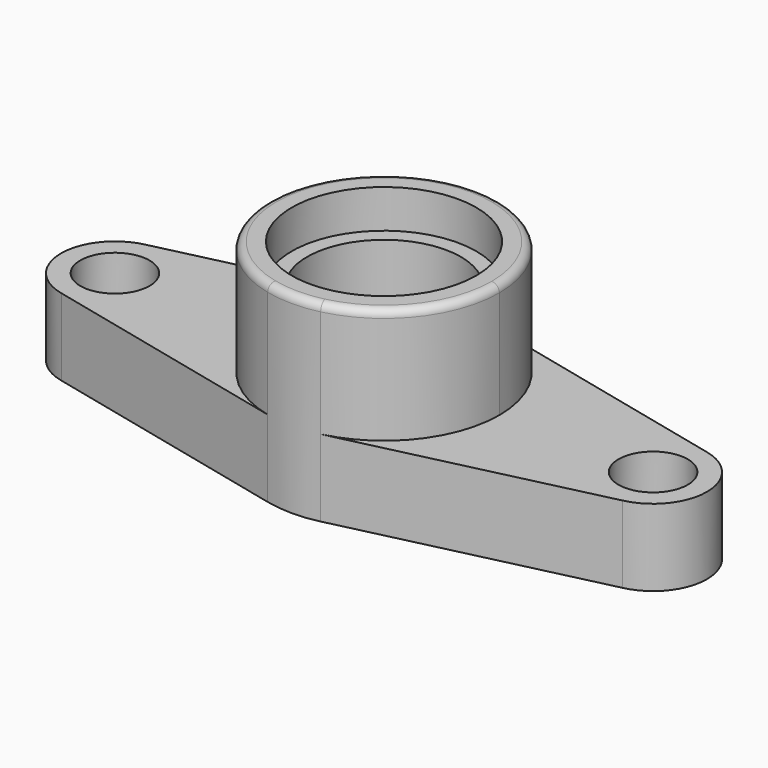
from build123d import *

# Parameters (mm, degrees)
F0_R     = 12
F0_R_2   = 4.5
F1_DEPTH = 10
F2_DEPTH = 25
F0_R_3   = 10
F3_DEPTH = 20
F0_R_4   = 3
F4_DEPTH = 5
F5_R     = 1


with BuildPart() as f1:
    # F0 (on Top) → F1 (new body)
    with BuildSketch(Plane.XY):
        with BuildLine():
            ThreePointArc((3.4443996306, -14.599181867), (11.761504888, -9.3095114142), (15, 0))
            ThreePointArc((15, 0), (11.761504888, 9.3095114142), (3.4443996306, 14.599181867))
            ThreePointArc((3.4443996306, 14.599181867), (0, 15), (-3.4443996306, 14.599181867))
            ThreePointArc((-3.4443996306, 14.599181867), (-15, 0), (-3.4443996306, -14.599181867))
            ThreePointArc((-3.4443996306, -14.599181867), (0, -15), (3.4443996306, -14.599181867))
        make_face()
        Circle(F0_R, mode=Mode.SUBTRACT)
        with BuildLine():
            ThreePointArc((3.4443996306, 14.599181867), (11.761504888, 9.3095114142), (15, 0))
            ThreePointArc((15, 0), (11.761504888, -9.3095114142), (3.4443996306, -14.599181867))
            Line((3.4443996306, -14.599181867), (36.4981958522, -6.8377927132))
            ThreePointArc((36.4981958522, -6.8377927132), (42, 0), (36.4981958522, 6.8377927132))
            Line((36.4981958522, 6.8377927132), (3.4443996306, 14.599181867))
        make_face()
        with Locations((35, 0)):
            Circle(F0_R_2, mode=Mode.SUBTRACT)
        with BuildLine():
            ThreePointArc((-3.4443996306, -14.599181867), (-15, 0), (-3.4443996306, 14.599181867))
            Line((-3.4443996306, 14.599181867), (-36.4981958522, 6.8377927132))
            ThreePointArc((-36.4981958522, 6.8377927132), (-42, 0), (-36.4981958522, -6.8377927132))
            Line((-36.4981958522, -6.8377927132), (-3.4443996306, -14.599181867))
        make_face()
        with Locations((-35, 0)):
            Circle(F0_R_2, mode=Mode.SUBTRACT)
    extrude(amount=F1_DEPTH)

    # F0 (on Top) → F4 (join)
    with BuildSketch(Plane.XY):
        with Locations((-35, 0)):
            Circle(F0_R_2)
        with Locations((-35, 0)):
            Circle(F0_R_4, mode=Mode.SUBTRACT)
        with Locations((35, 0)):
            Circle(F0_R_2)
        with Locations((35, 0)):
            Circle(F0_R_4, mode=Mode.SUBTRACT)
    extrude(amount=F4_DEPTH)


with BuildPart() as f2:
    # F0 (on Top) → F2 (new body)
    with BuildSketch(Plane.XY):
        with BuildLine():
            ThreePointArc((3.4443996306, -14.599181867), (11.761504888, -9.3095114142), (15, 0))
            ThreePointArc((15, 0), (11.761504888, 9.3095114142), (3.4443996306, 14.599181867))
            ThreePointArc((3.4443996306, 14.599181867), (0, 15), (-3.4443996306, 14.599181867))
            ThreePointArc((-3.4443996306, 14.599181867), (-15, 0), (-3.4443996306, -14.599181867))
            ThreePointArc((-3.4443996306, -14.599181867), (0, -15), (3.4443996306, -14.599181867))
        make_face()
        Circle(F0_R, mode=Mode.SUBTRACT)
    extrude(amount=F2_DEPTH)

    # F0 (on Top) → F3 (join)
    with BuildSketch(Plane.XY):
        Circle(F0_R)
        Circle(F0_R_3, mode=Mode.SUBTRACT)
    extrude(amount=F3_DEPTH)

    # F5
    f5_edges = [f2.edges().sort_by_distance(p)[0] for p in [
        (-3.4444, -14.599182, 25),
    ]]
    fillet(f5_edges, radius=F5_R)


solid = Compound([f1.part, f2.part])
